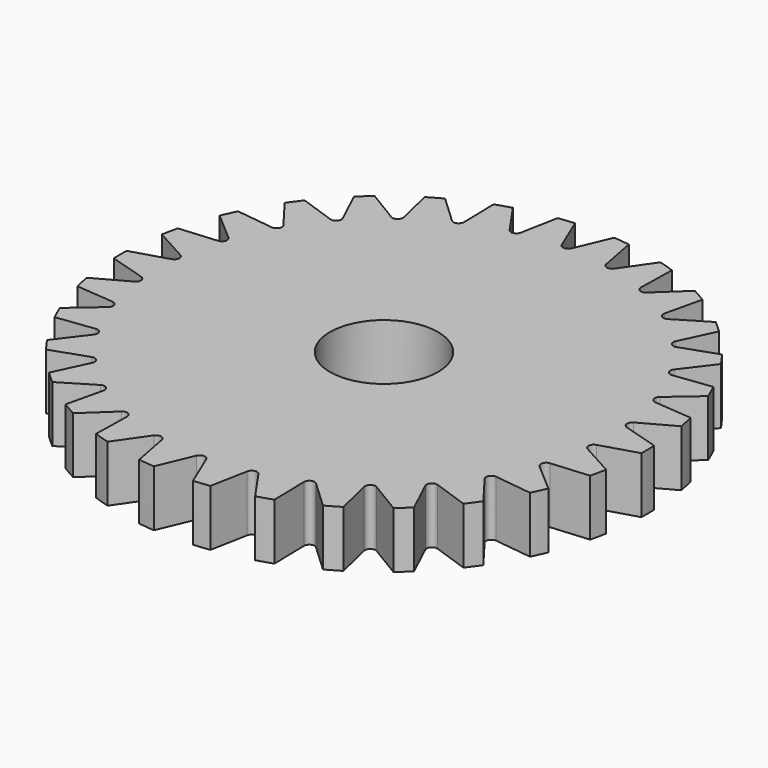
from build123d import *

# Parameters (mm, degrees)
F0_R            = 14.8770011714
F0_R_2          = 3.048
F1_DEPTH        = 3.175
F3_DEPTH        = 3.175
F3_COPIES_COUNT = 30


# Not quite as in the source:
# - a pattern or mirror of a feature is missing from the dataset's text; its kind, count and spacing are read off the source's solid


with BuildPart() as f1:
    # F0 (on Top) → F1 (new body)
    with BuildSketch(Plane.XY):
        Circle(F0_R)
        Circle(F0_R_2, mode=Mode.SUBTRACT)
    extrude(amount=F1_DEPTH)

    # F2 (on face) → F3 (cut, through all)
    with BuildSketch(Plane.XY.offset(3.175)):
        with BuildLine():
            Line((0.2742033495, 12.8709727929), (1.1020387684, 14.8361273386))
            ThreePointArc((1.1020387684, 14.8361273386), (0, 14.8770011714), (-1.1020387684, 14.8361273386))
            Line((-1.1020387684, 14.8361273386), (-0.2742033495, 12.8709727929))
            ThreePointArc((-0.2742033495, 12.8709727929), (0, 12.6889428931), (0.2742033495, 12.8709727929))
        make_face()
    f3 = extrude(amount=-F3_DEPTH, mode=Mode.SUBTRACT)

    # F3_copies: F3 ×30 about axis
    f3_copies_axis = Axis((0, 0, 0), (0, 0, 1))
    for i in range(1, F3_COPIES_COUNT):
        add(f3.rotate(f3_copies_axis, i * 360 / F3_COPIES_COUNT), mode=Mode.SUBTRACT)


solid = f1.part
